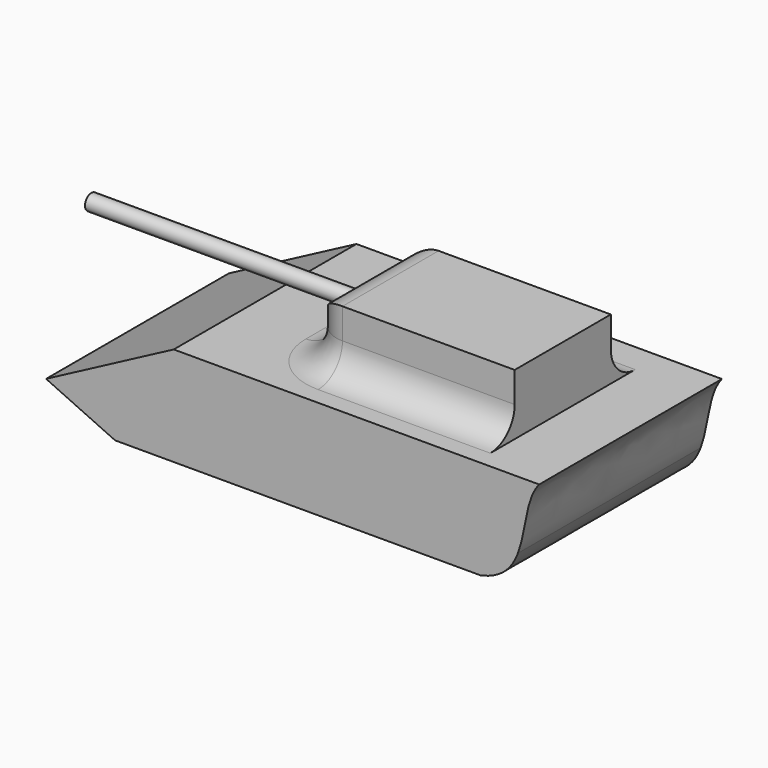
from build123d import *

# Parameters (mm, degrees)
F1_DEPTH = 38.1
F2_W     = 33.8070421275
F2_H     = 20.0418584555
F3_DEPTH = 10.16
F4_R     = 5.07999
F5_R     = 1.3208962066
F5_R_2   = 1.0238880826
F6_DEPTH = 60.96


# Not quite as in the source:
# - a fillet or chamfer is up to 0.001 mm smaller than in the source, because OpenCascade refuses the exact size
# - a feature names something its author has since deleted; it is built from what else it names


with BuildPart() as f1:
    # F0 (on Front) → F1 (new body)
    with BuildSketch(Plane.XZ):
        with BuildLine():
            Line((24.7568794588, -11.2399134781), (-53.9515846949, -11.2399134781))
            Line((-53.9515846949, -11.2399134781), (-42.4472021085, -16.5292843043))
            Line((-42.4472021085, -16.5292843043), (18.5127978915, -16.5292843043))
            add(Edge.make_bspline(
                [(18.5127978915, -16.5292843043), (22.1512323361, -15.7568533336), (23.817636294, -13.7140743109), (24.7568794588, -11.2399134781)],
                knots=[0, 0, 0, 0, 7.6693401108, 7.6693401108, 7.6693401108, 7.6693401108], degree=3))
        make_face()
        with BuildLine():
            Line((-32.6618658911, 0), (-53.9515846949, -11.2399134781))
            Line((-53.9515846949, -11.2399134781), (24.7568794588, -11.2399134781))
            add(Edge.make_bspline(
                [(24.7568794588, -11.2399134781), (26.1700602844, -7.5173027852), (25.9370894642, -2.8181269591), (28.2981341089, 0)],
                knots=[7.6693401108, 7.6693401108, 7.6693401108, 7.6693401108, 19.2085929859, 19.2085929859, 19.2085929859, 19.2085929859], degree=3))
            Line((28.2981341089, 0), (-32.6618658911, 0))
        make_face()
    extrude(amount=F1_DEPTH)

    # F2 (on Top) → F3 (join)
    with BuildSketch(Plane.XY):
        with Locations((0.9121662006, -20.0837139437)):
            Rectangle(F2_W, F2_H)
    extrude(amount=F3_DEPTH)

    # F4 (radius 5.08 in the source; OpenCascade refuses exactly that, so slightly less here)
    f4_edges = [f1.edges().sort_by_distance(p)[0] for p in [
        (-15.991355, -10.062785, 5.08),
        (-15.991355, -30.104643, 5.08),
        (-15.991355, -20.083714, 0),
        (-15.991355, -20.083714, 10.16),
        (0.912166, -30.104643, 0),
        (0.912166, -10.062785, 0),
    ]]
    fillet(f4_edges, radius=F4_R)

    # F5 (on Right) → F6 (join)
    with BuildSketch(Plane.YZ):
        with Locations((-19.9000276625, 5.0683720037)):
            Circle(F5_R)
        with Locations((-19.9000276625, 5.0683720037)):
            Circle(F5_R_2, mode=Mode.SUBTRACT)
    extrude(amount=-F6_DEPTH)


solid = f1.part
